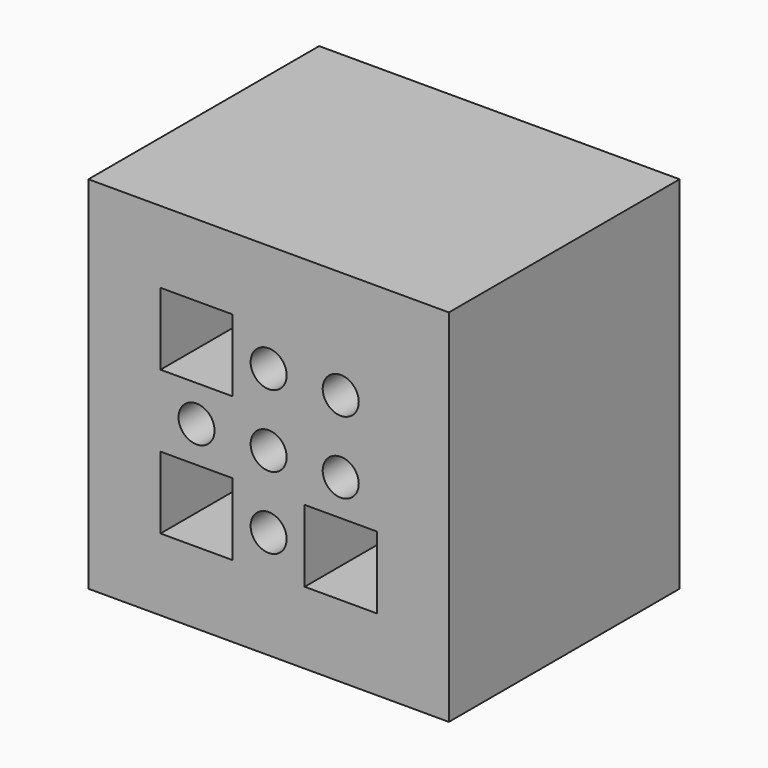
from build123d import *

# Parameters (mm, degrees)
F0_W     = 31.75
F0_H     = 31.75
F0_W_2   = 6.35
F0_H_2   = 6.35
F0_R     = 1.5875
F1_DEPTH = 25.4
F2_DEPTH = 3.175


# Not quite as in the source:
# - a length typed as a fraction of an inch, garbled in the dataset ("3 / 203.2 mm" for 3/8 in), is restored


with BuildPart() as f1:
    # F0 (on Front) → F1 (new body)
    with BuildSketch(Plane.XZ):
        with Locations((-5.7344107546, 14.0581134118)):
            Rectangle(F0_W, F0_H)
        with Locations((-12.0844107546, 7.7081134118)):
            Rectangle(F0_W_2, F0_H_2, mode=Mode.SUBTRACT)
        with Locations((-12.0844107546, 14.0581134118)):
            Circle(F0_R, mode=Mode.SUBTRACT)
        with Locations((-5.7344107546, 7.7081134118)):
            Circle(F0_R, mode=Mode.SUBTRACT)
        with Locations((0.6155892454, 7.7081134118)):
            Rectangle(F0_W_2, F0_H_2, mode=Mode.SUBTRACT)
        with Locations((-5.7344107546, 14.0581134118)):
            Circle(F0_R, mode=Mode.SUBTRACT)
        with Locations((0.6155892454, 14.0581134118)):
            Circle(F0_R, mode=Mode.SUBTRACT)
        with Locations((-12.0844107546, 20.4081134118)):
            Rectangle(F0_W_2, F0_H_2, mode=Mode.SUBTRACT)
        with Locations((-5.7344107546, 20.4081134118)):
            Circle(F0_R, mode=Mode.SUBTRACT)
        with Locations((0.6155892454, 20.4081134118)):
            Circle(F0_R, mode=Mode.SUBTRACT)
    extrude(amount=F1_DEPTH)

    # F0 (on Front) → F2 (join)
    with BuildSketch(Plane.XZ):
        with Locations((-5.7344107546, 14.0581134118)):
            Rectangle(F0_W, F0_H)
        with Locations((-12.0844107546, 7.7081134118)):
            Rectangle(F0_W_2, F0_H_2, mode=Mode.SUBTRACT)
        with Locations((-12.0844107546, 14.0581134118)):
            Circle(F0_R, mode=Mode.SUBTRACT)
        with Locations((-5.7344107546, 7.7081134118)):
            Circle(F0_R, mode=Mode.SUBTRACT)
        with Locations((0.6155892454, 7.7081134118)):
            Rectangle(F0_W_2, F0_H_2, mode=Mode.SUBTRACT)
        with Locations((-5.7344107546, 14.0581134118)):
            Circle(F0_R, mode=Mode.SUBTRACT)
        with Locations((0.6155892454, 14.0581134118)):
            Circle(F0_R, mode=Mode.SUBTRACT)
        with Locations((-12.0844107546, 20.4081134118)):
            Rectangle(F0_W_2, F0_H_2, mode=Mode.SUBTRACT)
        with Locations((-5.7344107546, 20.4081134118)):
            Circle(F0_R, mode=Mode.SUBTRACT)
        with Locations((0.6155892454, 20.4081134118)):
            Circle(F0_R, mode=Mode.SUBTRACT)
        with Locations((-12.0844107546, 7.7081134118)):
            Rectangle(F0_W_2, F0_H_2)
        with Locations((-5.7344107546, 7.7081134118)):
            Circle(F0_R)
        with Locations((0.6155892454, 7.7081134118)):
            Rectangle(F0_W_2, F0_H_2)
        with Locations((0.6155892454, 14.0581134118)):
            Circle(F0_R)
        with Locations((-5.7344107546, 14.0581134118)):
            Circle(F0_R)
        with Locations((-12.0844107546, 14.0581134118)):
            Circle(F0_R)
        with Locations((-12.0844107546, 20.4081134118)):
            Rectangle(F0_W_2, F0_H_2)
        with Locations((-5.7344107546, 20.4081134118)):
            Circle(F0_R)
        with Locations((0.6155892454, 20.4081134118)):
            Circle(F0_R)
    extrude(amount=F2_DEPTH)


solid = f1.part
